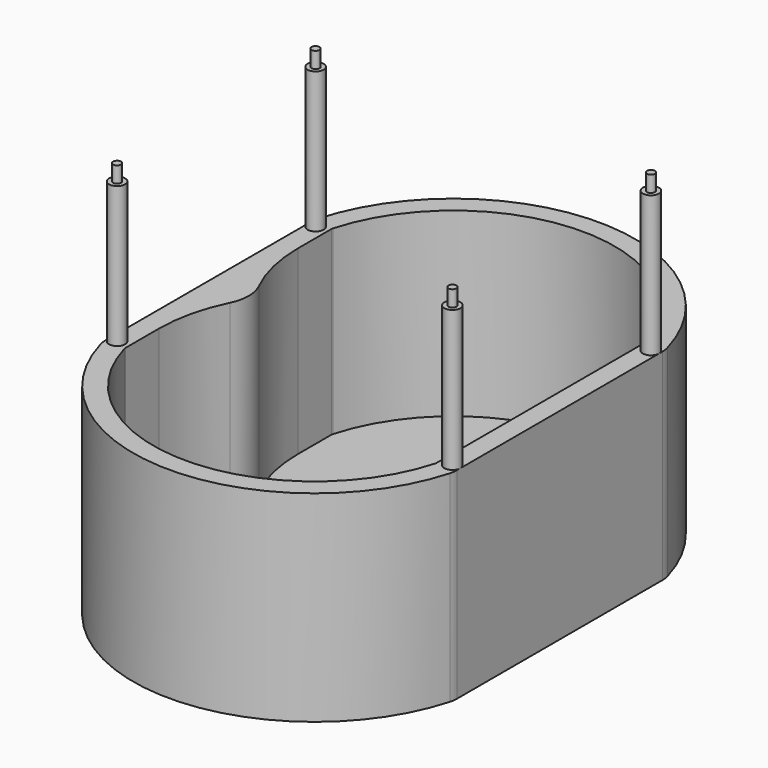
from build123d import *

# Parameters (mm, degrees)
F0_R     = 6
F1_DEPTH = 150
F2_T     = -15
F4_DEPTH = 135
F5_DEPTH = 105
F6_R     = 3
F7_DEPTH = 12


# Not quite as in the source:
# - a feature names something its author has since deleted; it is built from what else it names


with BuildPart() as f1:
    # F0 (on Top) → F1 (new body)
    with BuildSketch(Plane.XY):
        with BuildLine():
            Line((-131, -92.5), (-131, -95.859159479))
            ThreePointArc((-131, -95.859159479), (-130.8132026368, -98.5862460693), (-130.2562998729, -101.2623914012))
            ThreePointArc((-130.2562998729, -101.2623914012), (0, -200), (130.2562998729, -101.2623914012))
            ThreePointArc((130.2562998729, -101.2623914012), (130.8132026368, -98.5862460693), (131, -95.859159479))
            Line((131, -95.859159479), (131, -92.5))
            Line((131, -92.5), (131, 92.5))
            Line((131, 92.5), (131, 95.859159479))
            ThreePointArc((131, 95.859159479), (130.8132026368, 98.5862460693), (130.2562998729, 101.2623914012))
            ThreePointArc((130.2562998729, 101.2623914012), (0, 200), (-130.2562998729, 101.2623914012))
            ThreePointArc((-130.2562998729, 101.2623914012), (-130.8132026368, 98.5862460693), (-131, 95.859159479))
            Line((-131, 95.859159479), (-131, 92.5000001623))
            Line((-131, 92.5000001623), (-131, -92.5))
        make_face()
        with BuildLine():
            ThreePointArc((-119, -92.5), (-125, -98.5), (-131, -92.5))
            ThreePointArc((-131, -92.5), (-125, -86.5), (-119, -92.5))
        make_face(mode=Mode.SUBTRACT)
        with Locations((125, -92.5)):
            Circle(F0_R, mode=Mode.SUBTRACT)
        with BuildLine():
            ThreePointArc((-119, 92.5), (-125.0000000812, 86.5), (-131, 92.5000001623))
            ThreePointArc((-131, 92.5000001623), (-124.9999999188, 98.5), (-119, 92.5))
        make_face(mode=Mode.SUBTRACT)
        with Locations((125, 92.5)):
            Circle(F0_R, mode=Mode.SUBTRACT)
        with BuildLine():
            ThreePointArc((-119, -92.5), (-125, -86.5), (-131, -92.5))
            ThreePointArc((-131, -92.5), (-125, -98.5), (-119, -92.5))
        make_face()
        with BuildLine():
            ThreePointArc((-119, 92.5), (-124.9999999188, 98.5), (-131, 92.5000001623))
            ThreePointArc((-131, 92.5000001623), (-125.0000000812, 86.5), (-119, 92.5))
        make_face()
        with Locations((125, -92.5)):
            Circle(F0_R)
        with Locations((125, 92.5)):
            Circle(F0_R)
    extrude(amount=-F1_DEPTH)

    # F2
    f2_openings = [f1.faces().sort_by_distance(p)[0] for p in [
        (0, 0, 0),
    ]]
    offset(amount=F2_T, openings=f2_openings)

    # F3 (on face) → F4 (join, through all)
    with BuildSketch(Plane.XY):
        with BuildLine():
            ThreePointArc((-103.9827400965, 13.2972029152), (-112.95573879, 38.3122762743), (-116, 64.7130541872))
            Line((-116, 64.7130541872), (-116, -64.7130541872))
            ThreePointArc((-116, -64.7130541872), (-112.95573879, -38.3122762743), (-103.9827400965, -13.2972029152))
            ThreePointArc((-103.9827400965, -13.2972029152), (-100.8748280525, 0), (-103.9827400965, 13.2972029152))
        make_face()
    extrude(amount=-F4_DEPTH)

    # F0 (on Top) → F5 (join)
    with BuildSketch(Plane.XY):
        with Locations((125, -92.5)):
            Circle(F0_R)
        with Locations((125, 92.5)):
            Circle(F0_R)
        with BuildLine():
            ThreePointArc((-119, 92.5), (-124.9999999188, 98.5), (-131, 92.5000001623))
            ThreePointArc((-131, 92.5000001623), (-125.0000000812, 86.5), (-119, 92.5))
        make_face()
        with BuildLine():
            ThreePointArc((-119, -92.5), (-125, -86.5), (-131, -92.5))
            ThreePointArc((-131, -92.5), (-125, -98.5), (-119, -92.5))
        make_face()
    extrude(amount=F5_DEPTH)

    # F6 (on face) → F7 (join)
    with BuildSketch(Plane.XY.offset(105)):
        with Locations((125, -92.5)):
            Circle(F6_R)
        with Locations((-125, -92.5)):
            Circle(F6_R)
        with Locations((125, 92.5)):
            Circle(F6_R)
        with Locations((-125, 92.5)):
            Circle(F6_R)
    extrude(amount=F7_DEPTH)


solid = f1.part
